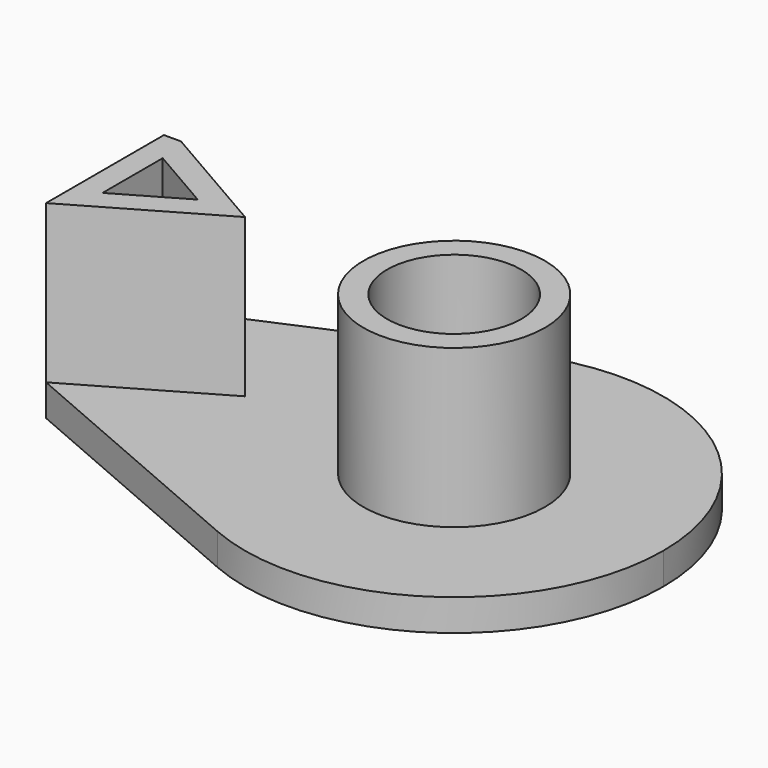
from build123d import *

# Parameters (mm, degrees)
F0_R     = 11.5
F0_R_2   = 8.5
F1_DEPTH = 4
F2_DEPTH = 20
F4_DEPTH = 10


# Not quite as in the source:
# - a feature names something its author has since deleted; it is built from what else it names


with BuildPart() as f1:
    # F0 (on Top) → F1 (new body)
    with BuildSketch(Plane.XY):
        Polygon((-43.75, -9.9592921435), (-26.5, 0), (-43.75, 9.9592921435), align=None)
        Polygon((-32.5, 0), (-40.75, -4.7631397208), (-40.75, 4.7631397208), align=None, mode=Mode.SUBTRACT)
        with BuildLine():
            Line((-43.75, 9.9592921435), (-26.5, 0))
            ThreePointArc((-26.5, 0), (-22.1457987188, 14.5538173379), (-10.514067992, 24.324974291))
            Line((-10.514067992, 24.324974291), (-43.75, 9.9592921435))
        make_face()
        with BuildLine():
            ThreePointArc((-10.514067992, 24.324974291), (-22.1457987188, 14.5538173379), (-26.5, 0))
            ThreePointArc((-26.5, 0), (-22.1457987188, -14.5538173379), (-10.514067992, -24.324974291))
            ThreePointArc((-10.514067992, -24.324974291), (14.5538173379, -22.1457987188), (26.5, 0))
            ThreePointArc((26.5, 0), (14.5538173379, 22.1457987188), (-10.514067992, 24.324974291))
        make_face()
        Circle(F0_R, mode=Mode.SUBTRACT)
        Circle(F0_R)
        Circle(F0_R_2, mode=Mode.SUBTRACT)
        with BuildLine():
            ThreePointArc((-10.514067992, -24.324974291), (-22.1457987188, -14.5538173379), (-26.5, 0))
            Line((-26.5, 0), (-43.75, -9.9592921435))
            Line((-43.75, -9.9592921435), (-10.514067992, -24.324974291))
        make_face()
    extrude(amount=-F1_DEPTH)

    # F0 (on Top) → F2 (join)
    with BuildSketch(Plane.XY):
        Polygon((-43.75, -9.9592921435), (-26.5, 0), (-43.75, 9.9592921435), align=None)
        Polygon((-32.5, 0), (-40.75, -4.7631397208), (-40.75, 4.7631397208), align=None, mode=Mode.SUBTRACT)
        Circle(F0_R)
        Circle(F0_R_2, mode=Mode.SUBTRACT)
    extrude(amount=F2_DEPTH)

    # F3 (on face) → F4 (cut)
    with BuildSketch(Plane(origin=(-43.75, 0, 0), x_dir=(0, -1, 0), z_dir=(-1, 0, 0))):
        Polygon((-9.9592921435, 1.25), (-9.9592921435, 0), (-8.7092921435, 0), align=None)
        Polygon((-9.9592921435, 3.75), (-9.9592921435, 1.25), (-8.7092921435, 2.5), align=None)
        Polygon((-8.7092921435, 5), (-9.9592921435, 6.25), (-9.9592921435, 3.75), align=None)
        Polygon((-8.7092921435, 7.5), (-9.9592921435, 8.75), (-9.9592921435, 6.25), align=None)
        Polygon((-8.7092921435, 10), (-9.9592921435, 11.25), (-9.9592921435, 8.75), align=None)
        Polygon((-8.7092921435, 12.5), (-9.9592921435, 13.75), (-9.9592921435, 11.25), align=None)
        Polygon((-8.7092921435, 15), (-9.9592921435, 16.25), (-9.9592921435, 13.75), align=None)
        Polygon((-8.7092921435, 17.5), (-9.9592921435, 18.75), (-9.9592921435, 16.25), align=None)
        Polygon((-9.9592921435, 18.75), (-8.7092921435, 20), (-9.9592921435, 20), align=None)
    extrude(amount=-F4_DEPTH, mode=Mode.SUBTRACT)


solid = f1.part
